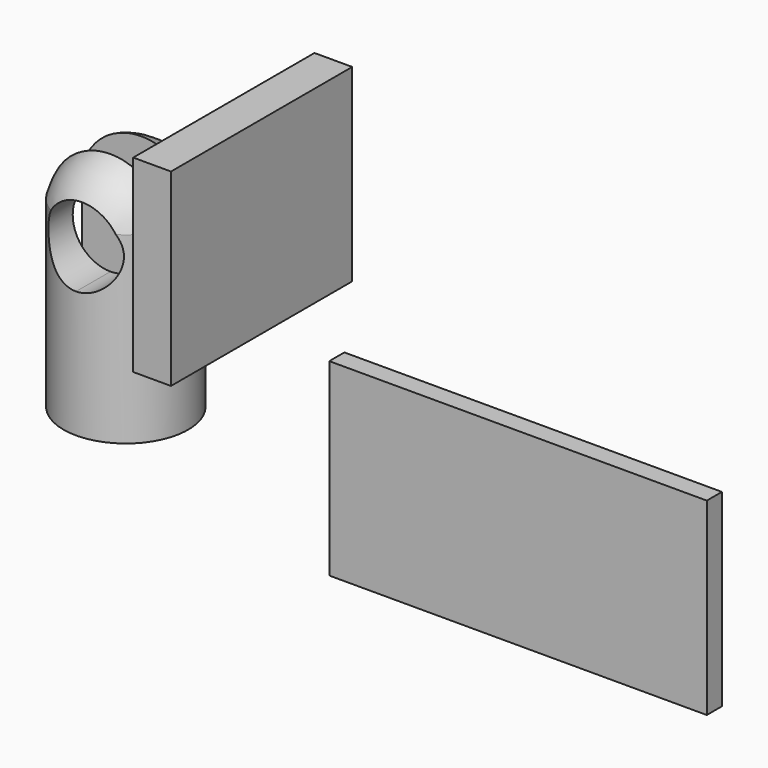
from build123d import *

# Parameters (mm, degrees)
F1_DEPTH = 6.35
F0_W     = 12.7
F0_H     = 63.5
F2_DEPTH = 76.2
F4_DEPTH = 20.9570915828
F5_DEPTH = 25.4
F6_W     = 41.9121831656
F6_H     = 12.954
F7_DEPTH = 78.4056


# Not quite as in the source:
# - a feature names something its author has since deleted; it is built from what else it names


with BuildPart() as f1:
    # F0 (on Front) → F1 (new body)
    with BuildSketch(Plane.XZ):
        Polygon((-32.8281914331, 8.6850252382), (-39.5913863666, 8.6850252382), (-39.5913863666, -54.8149747618), (-32.8281914331, -54.8149747618), (17.9718085669, -54.8149747618), (87.4086136334, -54.8149747618), (87.4086136334, 8.6850252382), (17.9718085669, 8.6850252382), align=None)
    extrude(amount=F1_DEPTH)


with BuildPart() as f2:
    # F0 (on Front) → F2 (new body)
    with BuildSketch(Plane.XZ):
        with Locations((-43.3035971761, 62.3321020156)):
            Rectangle(F0_W, F0_H)
    extrude(amount=F2_DEPTH)


with BuildPart() as f3:
    # F0 (on Front) → F3 (revolve)
    with BuildSketch(Plane.XZ):
        with BuildLine():
            ThreePointArc((-113.0859330297, 11.3450873971), (-125.7859330297, 24.0450873971), (-113.0859330297, 36.7450873971))
            Line((-113.0859330297, 36.7450873971), (-113.0859330297, 47.1505224705))
            ThreePointArc((-113.0859330297, 47.1505224705), (-126.4708775994, 42.47888537), (-134.0420246124, 30.4931160063))
            Line((-134.0420246124, 30.4931160063), (-134.0420246124, -31.3004925847))
            Line((-134.0420246124, -31.3004925847), (-113.0859330297, -31.3004925847))
            Line((-113.0859330297, -31.3004925847), (-113.0859330297, 11.3450873971))
        make_face()
        with BuildLine():
            ThreePointArc((-113.0859330297, 11.3450873971), (-104.1056769086, 15.064831276), (-100.3859330297, 24.0450873971))
            ThreePointArc((-100.3859330297, 24.0450873971), (-104.1056769086, 33.0253435182), (-113.0859330297, 36.7450873971))
            ThreePointArc((-113.0859330297, 36.7450873971), (-125.7859330297, 24.0450873971), (-113.0859330297, 11.3450873971))
        make_face()
    revolve(axis=Axis((-113.0859330297, 0, -9.9777025938), (0, 0, -1)))

    # F0 (on Front) → F4 (cut, through all)
    with BuildSketch(Plane.XZ):
        with BuildLine():
            ThreePointArc((-113.0859330297, 11.3450873971), (-104.1056769086, 15.064831276), (-100.3859330297, 24.0450873971))
            ThreePointArc((-100.3859330297, 24.0450873971), (-104.1056769086, 33.0253435182), (-113.0859330297, 36.7450873971))
            ThreePointArc((-113.0859330297, 36.7450873971), (-125.7859330297, 24.0450873971), (-113.0859330297, 11.3450873971))
        make_face()
    extrude(amount=-F4_DEPTH, mode=Mode.SUBTRACT)

    # F0 (on Front) → F5 (cut)
    with BuildSketch(Plane.XZ):
        with BuildLine():
            ThreePointArc((-113.0859330297, 11.3450873971), (-104.1056769086, 15.064831276), (-100.3859330297, 24.0450873971))
            ThreePointArc((-100.3859330297, 24.0450873971), (-104.1056769086, 33.0253435182), (-113.0859330297, 36.7450873971))
            ThreePointArc((-113.0859330297, 36.7450873971), (-125.7859330297, 24.0450873971), (-113.0859330297, 11.3450873971))
        make_face()
    extrude(amount=F5_DEPTH, mode=Mode.SUBTRACT)

    # F6 (on Top) → F7 (cut)
    with BuildSketch(Plane.XY):
        with Locations((-113.0859330297, 0)):
            Rectangle(F6_W, F6_H)
    extrude(amount=F7_DEPTH, mode=Mode.SUBTRACT)


solid = Compound([f1.part, f2.part, f3.part])
